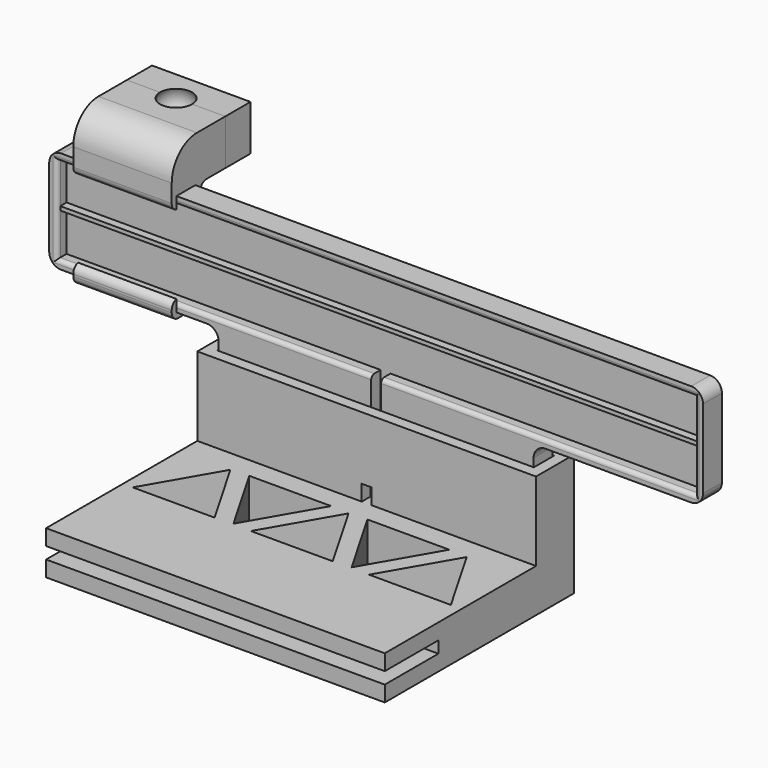
from build123d import *

# Parameters (mm, degrees)
F0_W              = 80
F0_H              = 25
F1_DEPTH          = 3
F3_DEPTH          = 3
F4_W              = 162
F4_H              = 1
F5_DEPTH          = 2
F6_R              = 3
F7_R              = 0.99999
F9_DEPTH          = 20
F10_W             = 85.9999992251
F10_H             = 11.9999992251
F11_DEPTH         = 2
F12_W             = 2.5
F12_H             = 4
F13_DEPTH         = 4
F14_W             = 85.9999992251
F14_H             = 60
F15_DEPTH         = 2
F17_DEPTH         = 3
F18_W             = 85.9999992251
F18_H             = 42.9999996126
F18_H_2           = 17.0000003874
F19_DEPTH         = 4
F21_DEPTH         = 50
F23_DEPTH         = 25
F25_W             = 25
F25_H             = 8.9999996647
F26_DEPTH         = 10
F27_W             = 25
F27_H             = 11.5619772188
F28_DEPTH         = 8
F31_W             = 25
F31_H             = 11.5619772188
F32_DEPTH         = 8
F34_R             = 8
F35_T1_DEPTH      = 25
F35_T3_DEPTH      = 34.6824581491
F35_T5_DEPTH      = 35
F35_T7_DEPTH      = 35
F35_T9_DEPTH      = 34.6824581491
F37_D             = 2.5
F37_DEPTH         = 13.5
F37_CSINK_D       = 6.72
F37_CSINK_ANGLE   = 90
F37_TIP           = 0.7510757738
F37_2_D           = 2.5
F37_2_DEPTH       = 13.5
F37_2_CSINK_D     = 6.72
F37_2_CSINK_ANGLE = 90
F37_2_TIP         = 0.7510757738
F38_D             = 3.3
F38_DEPTH         = 13.5
F38_CSINK_D       = 6.72
F38_CSINK_ANGLE   = 90
F38_TIP           = 0.9914200214


# Not quite as in the source:
# - a fillet or chamfer that OpenCascade refuses, or shapes differently, is made with other operations: its cross-section is extruded or revolved along the edge and cut away or added
# - a fillet or chamfer is up to 0.001 mm smaller than in the source, because OpenCascade refuses the exact size


with BuildPart() as f1:
    # F0 (on Front) → F1 (new body)
    with BuildSketch(Plane.XZ):
        Polygon((40, -13), (83, -13), (83, 13), (-83, 13), (-83, -13), (-40, -13), align=None)
        with Locations((0, -25.5)):
            Rectangle(F0_W, F0_H)
    extrude(amount=F1_DEPTH)

    # F2 (on face) → F3 (join)
    with BuildSketch(Plane.XZ.offset(3)):
        Polygon((83, -13), (83, 13), (-83, 13), (-83, -13), (-40, -13), (-40, -38), (-1.25, -38), (-1.25, -11), (-40, -11), (-81, -11), (-81, 11), (81, 11), (81, -11), (40, -11), (1.25, -11), (1.25, -38), (40, -38), (40, -13), align=None)
    extrude(amount=F3_DEPTH)

    # F4 (on face) → F5 (join)
    with BuildSketch(Plane.XZ.offset(3)):
        Rectangle(F4_W, F4_H)
    extrude(amount=F5_DEPTH)

    # F6
    f6_edges = [f1.edges().sort_by_distance(p)[0] for p in [
        (83, -3, 13),
        (83, -3, -13),
        (40, -3, -13),
        (-40, -3, -13),
        (-83, -3, -13),
        (-83, -3, 13),
        (40, -3, -38),
        (-40, -3, -38),
    ]]
    fillet(f6_edges, radius=F6_R)

    # F7 (radius 1 in the source; OpenCascade refuses exactly that, so slightly less here)
    f7_edges = [f1.edges().sort_by_distance(p)[0] for p in [
        (0, -6, 11),
        (-81, -6, 0),
        (-41.125, -6, -11),
        (41.125, -6, -11),
        (81, -6, 0),
    ]]
    fillet(f7_edges, radius=F7_R)


with BuildPart() as f9:
    # F8 (on face) → F9 (new body)
    with BuildSketch(Plane(origin=(0, 0, -38), x_dir=(1, 0, 0), z_dir=(0, 0, -1))):
        Polygon((37, 8.9999996126), (1.25, 8.9999996126), (-1.25, 8.9999996126), (-37, 8.9999996126), (-42.9999996126, 8.9999996126), (-42.9999996126, -2.9999996126), (-37, -2.9999996126), (37, -2.9999996126), (42.9999996126, -2.9999996126), (42.9999996126, 8.9999996126), align=None)
        Polygon((-40.2, 6.2), (-37, 6.2), (-1.25, 6.2), (1.25, 6.2), (37, 6.2), (40.2, 6.2), (40.2, -0.2), (37, -0.2), (-37, -0.2), (-40.2, -0.2), align=None, mode=Mode.SUBTRACT)
    extrude(amount=-F9_DEPTH)

    # F10 (on face) → F11 (join)
    with BuildSketch(Plane(origin=(0, 0, -38), x_dir=(1, 0, 0), z_dir=(0, 0, -1))):
        with Locations((0, 3)):
            Rectangle(F10_W, F10_H)
    extrude(amount=F11_DEPTH)

    # F12 (on face) → F13 (cut)
    with BuildSketch(Plane.XZ.offset(8.9999996126)):
        with Locations((0, -36)):
            Rectangle(F12_W, F12_H)
    extrude(amount=-F13_DEPTH, mode=Mode.SUBTRACT)

    # F14 (on face) → F15 (join, symmetric)
    with BuildSketch(Plane(origin=(0, 0, -40), x_dir=(1, 0, 0), z_dir=(0, 0, -1))):
        with Locations((0, 27.0000003874)):
            Rectangle(F14_W, F14_H)
    extrude(amount=F15_DEPTH, both=True)

    # F16 (on face) → F17 (join)
    with BuildSketch(Plane(origin=(0, 0, -42), x_dir=(1, 0, 0), z_dir=(0, 0, -1))):
        Polygon((-42.9999996126, 40), (-42.9999996126, 3.874e-07), (-42.9999996126, -2.9999996126), (42.9999996126, -2.9999996126), (42.9999996126, 0), (42.9999996126, 40), align=None)
    extrude(amount=F17_DEPTH)

    # F18 (on face) → F19 (join)
    with BuildSketch(Plane(origin=(0, 0, -45), x_dir=(1, 0, 0), z_dir=(0, 0, -1))):
        with Locations((0, 18.5000001937)):
            Rectangle(F18_W, F18_H)
        with Locations((0, 48.5000001937)):
            Rectangle(F18_W, F18_H_2)
    extrude(amount=F19_DEPTH)

    # F20 (on face) → F21 (cut)
    with BuildSketch(Plane.XY.offset(-38)):
        Polygon((-40.527221151, -32.5934187919), (-19.7426114601, -32.5934187919), (-30.1349163055, -14.5934187919), align=None)
        Polygon((-10.527221151, -32.5934187919), (10.2573885399, -32.5934187919), (-0.1349163055, -14.5934187919), align=None)
        Polygon((19.472778849, -32.5934187919), (40.2573885399, -32.5934187919), (29.8650836945, -14.5934187919), align=None)
        Polygon((-4.8039347303, -14.2831178904), (-25.5885444212, -14.2831178904), (-15.1962395757, -32.2831178904), align=None)
        Polygon((25.1960652697, -14.2831178904), (4.4114555788, -14.2831178904), (14.8037604243, -32.2831178904), align=None)
    extrude(amount=-F21_DEPTH, mode=Mode.SUBTRACT)


with BuildPart() as f23:
    # F22 (on Right) → F23 (new body)
    with BuildSketch(Plane.YZ):
        Polygon((-6, 13), (0, 13), (0, 10), (0, -10), (0, -13), (-6, -13), (-6, -10), (-7.4999998324, -10), (-7.4999998324, -14.4999998324), (1.4999998324, -14.4999998324), (1.4999998324, -10), (1.4999998324, 10), (1.4999998324, 14.4999998324), (-7.4999998324, 14.4999998324), (-7.4999998324, 10), (-6, 10), align=None)
    extrude(amount=F23_DEPTH)


with BuildPart() as f23_1:
    # F24: moved
    add(f23.part.moved(Location((-75.7, 0, 0))))

    # F25 (on face) → F26 (join)
    with BuildSketch(Plane.XY.offset(14.4999998324)):
        with Locations((-63.2, -3)):
            Rectangle(F25_W, F25_H)
    extrude(amount=F26_DEPTH)

    # F27 (on face) → F28 (join)
    with BuildSketch(Plane(origin=(0, 1.4999998324, 0), x_dir=(-1, 0, 0), z_dir=(0, 1, 0))):
        with Locations((63.2, 18.7190112229)):
            Rectangle(F27_W, F27_H)
    extrude(amount=F28_DEPTH)


with BuildPart() as f30:
    # F29 (on face) → F30 (revolve)
    with BuildSketch(Plane(origin=(0, 9.4999998324, 0), x_dir=(-1, 0, 0), z_dir=(0, 1, 0))):
        with BuildLine():
            Line((63.2, 24.4999998324), (63.2, 16.6022711247))
            ThreePointArc((63.2, 16.6022711247), (67.6434583118, 19.3097445205), (67.2746985578, 24.4999998324))
            Line((67.2746985578, 24.4999998324), (63.2, 24.4999998324))
        make_face()
    revolve(axis=Axis((-63.2, 9.4999998324, 21.6022711247), (0, 0, 1)))


with BuildPart() as f32:
    # F31 (on face) → F32 (new body)
    with BuildSketch(Plane(origin=(0, 9.4999998324, 0), x_dir=(-1, 0, 0), z_dir=(0, 1, 0))):
        with Locations((63.2, 18.7190112229)):
            Rectangle(F31_W, F31_H)
    extrude(amount=F32_DEPTH)

    # F33: cut F30
    add(f30.part, mode=Mode.SUBTRACT)

    # F37#2
    with Locations(Plane(origin=(0, 17.4999998324, 0), x_dir=(-1, 0, 0), z_dir=(0, 1, 0))):
        with Locations((54.2, 18.7190112229), (72.2, 18.7190112229)):
            CounterSinkHole(F37_2_D / 2, F37_2_CSINK_D / 2, depth=F37_2_DEPTH, counter_sink_angle=F37_2_CSINK_ANGLE)
            with Locations((0, 0, -(F37_2_DEPTH + F37_2_TIP / 2))):  # 118° drill point
                Cone(0, F37_2_D / 2, F37_2_TIP, mode=Mode.SUBTRACT)

    # F38
    with Locations(Plane(origin=(0, 17.4999998324, 0), x_dir=(-1, 0, 0), z_dir=(0, 1, 0))):
        with Locations((54.2, 18.7190112229), (72.2, 18.7190112229)):
            CounterSinkHole(F38_D / 2, F38_CSINK_D / 2, depth=F38_DEPTH, counter_sink_angle=F38_CSINK_ANGLE)
            with Locations((0, 0, -(F38_DEPTH + F38_TIP / 2))):  # 118° drill point
                Cone(0, F38_D / 2, F38_TIP, mode=Mode.SUBTRACT)


with BuildPart() as f23_2:
    add(f23_1.part)

    # F33: cut F30
    add(f30.part, mode=Mode.SUBTRACT)

    # F34
    f34_edges = [f23_2.edges().sort_by_distance(p)[0] for p in [
        (-63.2, -7.5, 24.5),
    ]]
    fillet(f34_edges, radius=F34_R)

    # F35: fillet of radius 2 on 5 edges, made by hand

    # F35_s2 → F35_t1 (join)
    with BuildSketch(Plane.YZ.offset(-75.7)):
        with BuildLine():
            ThreePointArc((3.4999998324, 12.9380226135), (2.08578627, 12.3522361759), (1.4999998324, 10.9380226135))
            Line((1.4999998324, 10.9380226135), (1.4999998324, 12.9380226135))
            Line((1.4999998324, 12.9380226135), (3.4999998324, 12.9380226135))
        make_face()
    extrude(amount=F35_T1_DEPTH)

    # F35_s4 → F35_t3 (cut)
    with BuildSketch(Plane.YZ.offset(-80.5412290745)):
        with BuildLine():
            ThreePointArc((-7.4999998324, 11.9364916298), (-7.0811387155, 10.7117468269), (-6, 10))
            Line((-6, 10), (-7.4999998324, 10))
            Line((-7.4999998324, 10), (-7.4999998324, 11.9364916298))
        make_face()
    extrude(amount=F35_T3_DEPTH, mode=Mode.SUBTRACT)

    # F35_s6 → F35_t5 (cut)
    with BuildSketch(Plane.YZ.offset(-80.7)):
        with BuildLine():
            ThreePointArc((1.4999998324, -12.4999998324), (0.9142133947, -13.9142133947), (-0.5000001676, -14.4999998324))
            Line((-0.5000001676, -14.4999998324), (1.4999998324, -14.4999998324))
            Line((1.4999998324, -14.4999998324), (1.4999998324, -12.4999998324))
        make_face()
    extrude(amount=F35_T5_DEPTH, mode=Mode.SUBTRACT)

    # F35_s8 → F35_t7 (cut)
    with BuildSketch(Plane.YZ.offset(-80.7)):
        with BuildLine():
            ThreePointArc((-5.4999998324, -14.4999998324), (-6.9142133947, -13.9142133947), (-7.4999998324, -12.4999998324))
            Line((-7.4999998324, -12.4999998324), (-7.4999998324, -14.4999998324))
            Line((-7.4999998324, -14.4999998324), (-5.4999998324, -14.4999998324))
        make_face()
    extrude(amount=F35_T7_DEPTH, mode=Mode.SUBTRACT)

    # F35_s10 → F35_t9 (cut)
    with BuildSketch(Plane.YZ.offset(-80.5412290745)):
        with BuildLine():
            ThreePointArc((-7.4999998324, -11.9364916298), (-7.0811387155, -10.7117468269), (-6, -10))
            Line((-6, -10), (-7.4999998324, -10))
            Line((-7.4999998324, -10), (-7.4999998324, -11.9364916298))
        make_face()
    extrude(amount=F35_T9_DEPTH, mode=Mode.SUBTRACT)

    # F37
    with Locations(Plane(origin=(0, 17.4999998324, 0), x_dir=(-1, 0, 0), z_dir=(0, 1, 0))):
        with Locations((54.2, 18.7190112229), (72.2, 18.7190112229)):
            CounterSinkHole(F37_D / 2, F37_CSINK_D / 2, depth=F37_DEPTH, counter_sink_angle=F37_CSINK_ANGLE)
            with Locations((0, 0, -(F37_DEPTH + F37_TIP / 2))):  # 118° drill point
                Cone(0, F37_D / 2, F37_TIP, mode=Mode.SUBTRACT)


solid = Compound([f1.part, f9.part, f32.part, f23_2.part])
